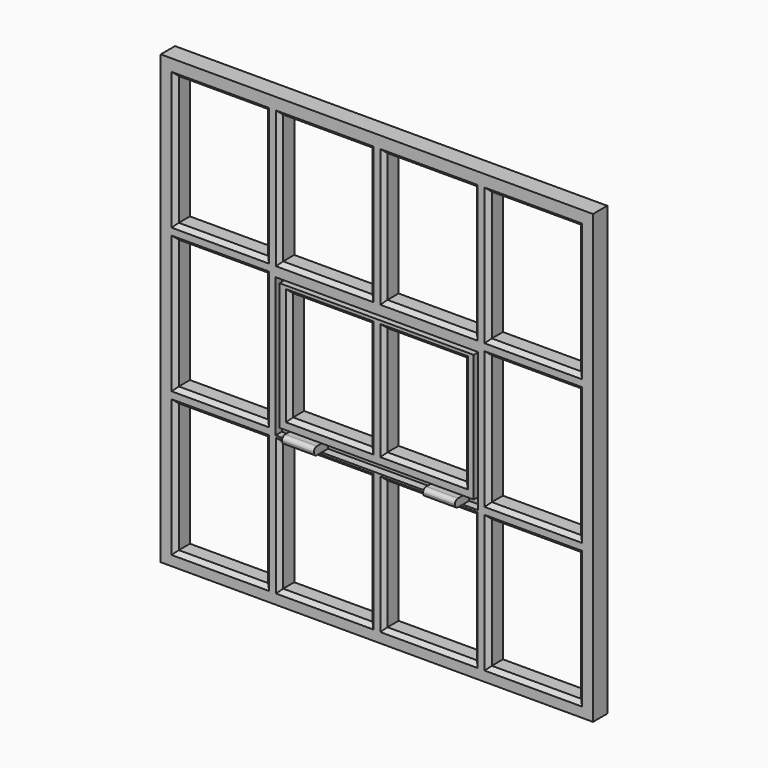
from build123d import *

# Parameters (mm, degrees)
F0_W     = 9
F0_H     = 13
F1_DEPTH = 1.8
F2_DEPTH = 1
F3_DEPTH = 1
F4_DEPTH = 1
F5_DEPTH = 1
F7_DEPTH = 0.8
F8_W     = 3.2
F8_H     = 0.8
F9_DEPTH = 1
F10_R    = 0.39999
F11_SIZE = 0.4


# Not quite as in the source:
# - a fillet or chamfer is up to 0.001 mm smaller than in the source, because OpenCascade refuses the exact size
# - a feature names something its author has since deleted; it is built from what else it names


with BuildPart() as f1:
    # F0 (on Front) → F1 (new body)
    with BuildSketch(Plane.XZ):
        Polygon((-22, -22.5), (21.5, -22.5), (21.5, 22.5), (-22, 22.5), (-22, -7.5), align=None)
        with Locations((-16, -14.6)):
            Rectangle(F0_W, F0_H, mode=Mode.SUBTRACT)
        with Locations((-5.5, -14.6)):
            Rectangle(F0_W, F0_H, mode=Mode.SUBTRACT)
        with Locations((-16, -0.1)):
            Rectangle(F0_W, F0_H, mode=Mode.SUBTRACT)
        with Locations((-5.5, -0.1)):
            Rectangle(F0_W, F0_H, mode=Mode.SUBTRACT)
        with Locations((5, -14.6)):
            Rectangle(F0_W, F0_H, mode=Mode.SUBTRACT)
        with Locations((15.5, -14.6)):
            Rectangle(F0_W, F0_H, mode=Mode.SUBTRACT)
        with Locations((5, -0.1)):
            Rectangle(F0_W, F0_H, mode=Mode.SUBTRACT)
        with Locations((15.5, -0.1)):
            Rectangle(F0_W, F0_H, mode=Mode.SUBTRACT)
        with Locations((-16, 14.4)):
            Rectangle(F0_W, F0_H, mode=Mode.SUBTRACT)
        with Locations((-5.5, 14.4)):
            Rectangle(F0_W, F0_H, mode=Mode.SUBTRACT)
        with Locations((5, 14.4)):
            Rectangle(F0_W, F0_H, mode=Mode.SUBTRACT)
        with Locations((15.5, 14.4)):
            Rectangle(F0_W, F0_H, mode=Mode.SUBTRACT)
    extrude(amount=F1_DEPTH)

    # F2 (add): a face of the model
    f2_faces = [f1.faces().sort_by_distance(p)[0] for p in [
        (9.5, -0.9, -0.1),
    ]]
    extrude(f2_faces, amount=F2_DEPTH)

    # F3 (add): a face of the model
    f3_faces = [f1.faces().sort_by_distance(p)[0] for p in [
        (-10, -0.9, -0.1),
    ]]
    extrude(f3_faces, amount=F3_DEPTH)

    # F4 (add): faces of the model
    f4_faces = [f1.faces().sort_by_distance(p)[0] for p in [
        (-5, -0.9, 6.4),
        (4.5, -0.9, 6.4),
    ]]
    extrude(f4_faces, amount=F4_DEPTH)

    # F5 (add): faces of the model
    f5_faces = [f1.faces().sort_by_distance(p)[0] for p in [
        (-5, -0.9, -6.6),
        (4.5, -0.9, -6.6),
    ]]
    extrude(f5_faces, amount=F5_DEPTH)

    # F6 (on face) → F7 (cut)
    with BuildSketch(Plane.XZ.offset(1.8)):
        Polygon((5.2, -7.5), (5.2, -6.7), (-5.8, -6.7), (-5.8, -7.5), (-0.25, -7.5), align=None)
        Polygon((-9, -6.7), (-10.05, -6.7), (-10.45, -6.7), (-10.45, -7.5), (-9, -7.5), align=None)
        Polygon((9.5, 6.1155543663), (9.5, -6.7), (8.4, -6.7), (8.4, -7.5), (9.95, -7.5), (9.95, 6.5155543663), (-10.45, 6.5155543663), (-10.45, -6.7), (-10.05, -6.7), (-10.05, 6.1155543663), align=None)
    extrude(amount=-F7_DEPTH, mode=Mode.SUBTRACT)

    # F8 (on face) → F9 (join)
    with BuildSketch(Plane.XZ.offset(1.8)):
        with Locations((6.8, -7.1)):
            Rectangle(F8_W, F8_H)
        with Locations((-7.4, -7.1)):
            Rectangle(F8_W, F8_H)
    extrude(amount=F9_DEPTH)

    # F10 (radius 0.4 in the source; OpenCascade refuses exactly that, so slightly less here)
    f10_edges = [f1.edges().sort_by_distance(p)[0] for p in [
        (6.8, -2.8, -6.7),
        (6.8, -2.8, -7.5),
        (-7.4, -2.8, -7.5),
        (-7.4, -2.8, -6.7),
    ]]
    fillet(f10_edges, radius=F10_R)

    # F11
    f11_edges = [f1.edges().sort_by_distance(p)[0] for p in [
        (-20.5, -1.8, 14.4),
        (-11.5, -1.8, 14.4),
        (-16, -1.8, 20.9),
        (-16, -1.8, 7.9),
        (-16, -1.8, 6.4),
        (-20.5, -1.8, -0.1),
        (-16, -1.8, -6.6),
        (-11.5, -1.8, -0.1),
        (-5.5, -1.8, 7.9),
        (-10, -1.8, 14.4),
        (-1, -1.8, 14.4),
        (0.5, -1.8, 14.4),
        (5, -1.8, 7.9),
        (9.5, -1.8, 14.4),
        (-5, -1.8, 5.4),
        (-9, -1.8, -0.1),
        (-1, -1.8, -0.1),
        (0.5, -1.8, -0.1),
        (4.5, -1.8, 5.4),
        (8.5, -1.8, -0.1),
        (4.5, -1.8, -5.6),
        (-5, -1.8, -5.6),
        (-5.5, -1.8, 20.9),
        (5, -1.8, 20.9),
        (15.5, -1.8, 20.9),
        (20, -1.8, 14.4),
        (15.5, -1.8, 7.9),
        (11, -1.8, 14.4),
        (15.5, -1.8, 6.4),
        (11, -1.8, -0.1),
        (20, -1.8, -0.1),
        (15.5, -1.8, -6.6),
        (15.5, -1.8, -8.1),
        (11, -1.8, -14.6),
        (15.5, -1.8, -21.1),
        (20, -1.8, -14.6),
        (9.5, -1.8, -14.6),
        (5, -1.8, -8.1),
        (0.5, -1.8, -14.6),
        (5, -1.8, -21.1),
        (-5.5, -1.8, -21.1),
        (-1, -1.8, -14.6),
        (-5.5, -1.8, -8.1),
        (-10, -1.8, -14.6),
        (-11.5, -1.8, -14.6),
        (-16, -1.8, -8.1),
        (-20.5, -1.8, -14.6),
        (-16, -1.8, -21.1),
    ]]
    chamfer(f11_edges, length=F11_SIZE)


solid = f1.part
